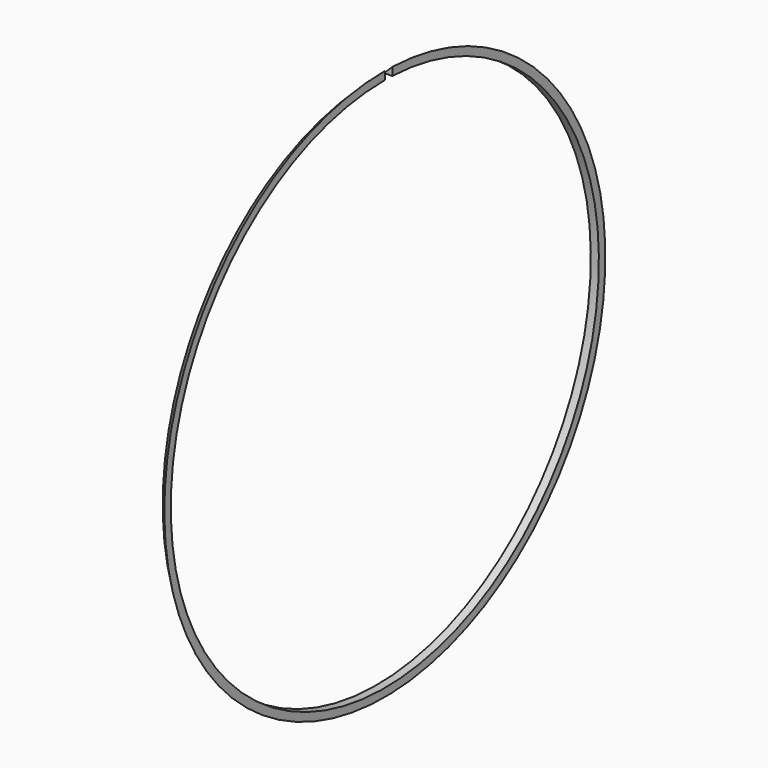
from build123d import *

# Parameters (mm, degrees)
F0_W     = 2.54
F0_H     = 2.54
F2_ANGLE = 358
F3_SIZE  = 2.53999


# Not quite as in the source:
# - a fillet or chamfer is up to 0.001 mm smaller than in the source, because OpenCascade refuses the exact size


with BuildPart() as f2:
    # F0 (on Front) → F2 (revolve)
    with BuildSketch(Plane.XZ):
        with Locations((-7.6375972124, 85.4075)):
            Rectangle(F0_W, F0_H)
    revolve(axis=Axis((5.7470723987, 0, 0), (1, 0, 0)), revolution_arc=F2_ANGLE)

    # F3 (size 2.54 in the source; OpenCascade refuses exactly that, so slightly less here)
    f3_edges = [f2.edges().sort_by_distance(p)[0] for p in [
        (-8.907597, -1.512731, -86.664299),
    ]]
    chamfer(f3_edges, length=F3_SIZE)


solid = f2.part
